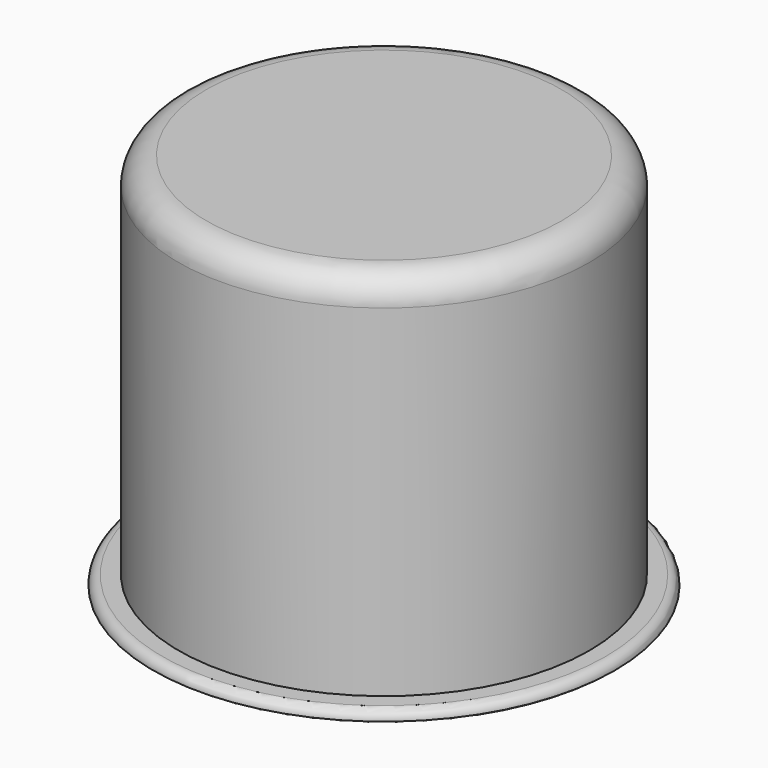
from build123d import *

# Parameters (mm, degrees)
F0_R     = 56.515
F1_DEPTH = 101.6
F2_R     = 52.07
F3_DEPTH = 95.25
F4_R     = 63.5
F5_DEPTH = 3.175
F6_R     = 52.07
F7_DEPTH = 12.7
F8_R     = 7.62
F9_R     = 2.54
F10_R    = 2.54


# Not quite as in the source:
# - a fillet or chamfer that OpenCascade refuses, or shapes differently, is made with other operations: its cross-section is extruded or revolved along the edge and cut away or added


with BuildPart() as f1:
    # F0 (on Top) → F1 (new body)
    with BuildSketch(Plane.XY):
        Circle(F0_R)
    extrude(amount=F1_DEPTH)

    # F2 (on Top) → F3 (cut)
    with BuildSketch(Plane.XY):
        Circle(F2_R)
    extrude(amount=F3_DEPTH, mode=Mode.SUBTRACT)

    # F4 (on face) → F5 (join)
    with BuildSketch(Plane(origin=(0, 0, 0), x_dir=(1, 0, 0), z_dir=(0, 0, -1))):
        Circle(F4_R)
    extrude(amount=F5_DEPTH)

    # F6 (on Top) → F7 (cut)
    with BuildSketch(Plane.XY):
        Circle(F6_R)
    extrude(amount=-F7_DEPTH, mode=Mode.SUBTRACT)

    # F8
    f8_edges = [f1.edges().sort_by_distance(p)[0] for p in [
        (-56.515, 0, 101.6),
    ]]
    fillet(f8_edges, radius=F8_R)

    # F9
    f9_edges = [f1.edges().sort_by_distance(p)[0] for p in [
        (-52.07, 0, -3.175),
    ]]
    fillet(f9_edges, radius=F9_R)

    # F10
    f10_edges = [f1.edges().sort_by_distance(p)[0] for p in [
        (-63.5, 0, 0),
    ]]
    fillet(f10_edges, radius=F10_R)

    # F11: fillet of radius 2.54 on 1 edges, made by hand

    # F11_s1 → F11_t2 (revolve, cut)
    with BuildSketch(Plane.XZ):
        with BuildLine():
            ThreePointArc((63.5, -2.54), (62.7179735296, -3.0109524406), (61.8199479175, -3.175))
            Line((61.8199479175, -3.175), (63.5, -3.175))
            Line((63.5, -3.175), (63.5, -2.54))
        make_face()
    revolve(axis=Axis((0, 0, -3.175), (0, 0, -1)), mode=Mode.SUBTRACT)


solid = f1.part
